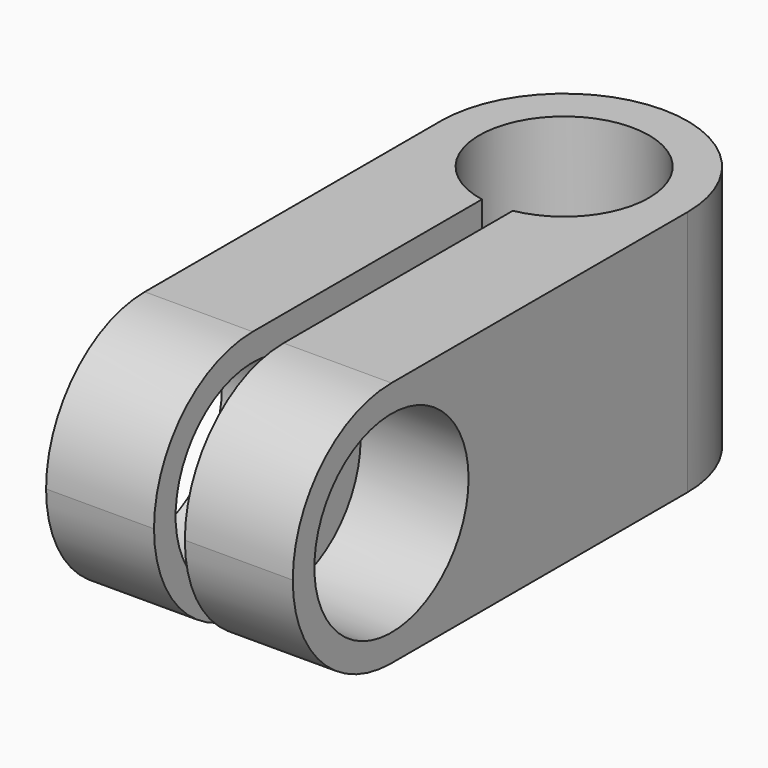
from build123d import *

# Parameters (mm, degrees)
F0_W      = 8
F0_H      = 8
F1_DEPTH  = 20
F3_DEPTH  = 15
F4_R      = 3.99999
F6_DEPTH  = 10
F7_R      = 3.125
F8_DEPTH  = 8.001
F9_DEPTH  = 25
F10_DEPTH = 27


# Not quite as in the source:
# - a fillet or chamfer is up to 0.001 mm smaller than in the source, because OpenCascade refuses the exact size


with BuildPart() as f1:
    # F0 (on Front) → F1 (new body)
    with BuildSketch(Plane.XZ):
        with Locations((4, 4)):
            Rectangle(F0_W, F0_H)
    extrude(amount=F1_DEPTH)

    # F2 (on face) → F3 (cut)
    with BuildSketch(Plane.XZ.offset(20)):
        Polygon((4.5, 8), (4, 8), (3.5, 8), (3.5, 0), (4.5, 0), align=None)
    extrude(amount=-F3_DEPTH, mode=Mode.SUBTRACT)

    # F4 (radius 4 in the source; OpenCascade refuses exactly that, so slightly less here)
    f4_edges = [f1.edges().sort_by_distance(p)[0] for p in [
        (1.75, -20, 8),
        (6.25, -20, 8),
        (6.25, -20, 0),
        (1.75, -20, 0),
        (8, 0, 4),
        (0, 0, 4),
    ]]
    fillet(f4_edges, radius=F4_R)

    # F5 (on face) → F6 (join)
    with BuildSketch(Plane.XY.offset(8)):
        with BuildLine():
            Line((3.5, -5), (3.5, -6.7041634566))
            ThreePointArc((3.5, -6.7041634566), (4, -6.75), (4.5, -6.7041634566))
            Line((4.5, -6.7041634566), (4.5, -5))
            Line((4.5, -5), (3.5, -5))
        make_face()
        with BuildLine():
            ThreePointArc((4.5, -6.7041634566), (6.1139418157, -5.7589059099), (6.75, -4))
            ThreePointArc((6.75, -4), (2.2410940901, -1.8860581843), (3.5, -6.7041634566))
            Line((3.5, -6.7041634566), (3.5, -5))
            Line((3.5, -5), (4.5, -5))
            Line((4.5, -5), (4.5, -6.7041634566))
        make_face()
    extrude(amount=-F6_DEPTH)

    # F7 (on face) → F8 (join, through all)
    with BuildSketch(Plane.YZ.offset(8)):
        with Locations((-16, 4)):
            Circle(F7_R)
    extrude(amount=-F8_DEPTH)

    # F9 (cut): a face of the model
    f9_faces = [f1.faces().sort_by_distance(p)[0] for p in [
        (4, -4, -2),
    ]]
    extrude(f9_faces, amount=-F9_DEPTH, mode=Mode.SUBTRACT)

    # F10 (cut): a face of the model
    f10_faces = [f1.faces().sort_by_distance(p)[0] for p in [
        (-0.001, -16, 4),
    ]]
    extrude(f10_faces, amount=-F10_DEPTH, mode=Mode.SUBTRACT)


solid = f1.part
